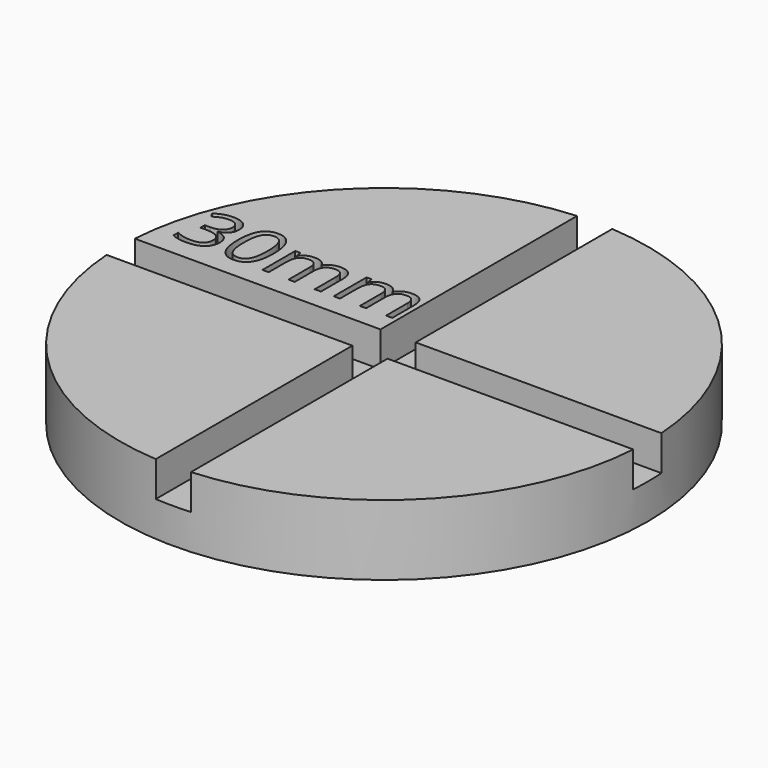
from build123d import *

# Parameters (mm, degrees)
F0_R         = 15
F1_DEPTH     = 4
F2_W         = 23.6895670906
F2_H         = 2
F2_W_2       = 2
F2_H_2       = 16.6301561296
F3_DEPTH     = 2
F4_TEXT_SIZE = 4.358786246
F5_DEPTH     = 1


# Not quite as in the source:
# - Text() gives the source's letters only with a copy of the font that has no kerning and outlines rounded to 1/6400 em; it was checked with that copy


with BuildPart() as f1:
    # F0 (on Top) → F1 (new body)
    with BuildSketch(Plane.XY):
        Circle(F0_R)
    extrude(amount=F1_DEPTH)

    # F2 (on face) → F3 (cut)
    with BuildSketch(Plane.XY.offset(4)):
        with Locations((12.8447835453, 0)):
            Rectangle(F2_W, F2_H)
        with Locations((0, -9.3150780648)):
            Rectangle(F2_W_2, F2_H_2)
        Rectangle(F2_W_2, F2_H)
        with Locations((-12.8447835453, 0)):
            Rectangle(F2_W, F2_H)
        with Locations((0, 9.3150780648)):
            Rectangle(F2_W_2, F2_H_2)
    extrude(amount=-F3_DEPTH, mode=Mode.SUBTRACT)

    # F4 (on face) → F5 (cut)
    with BuildSketch(Plane.XY.offset(4)):
        with Locations((-14.0218739098, 2.1896239831)):
            Text('30mm', F4_TEXT_SIZE, font='Open Sans', text_align=(TextAlign.LEFT, TextAlign.BOTTOM))
    extrude(amount=-F5_DEPTH, mode=Mode.SUBTRACT)


solid = f1.part
